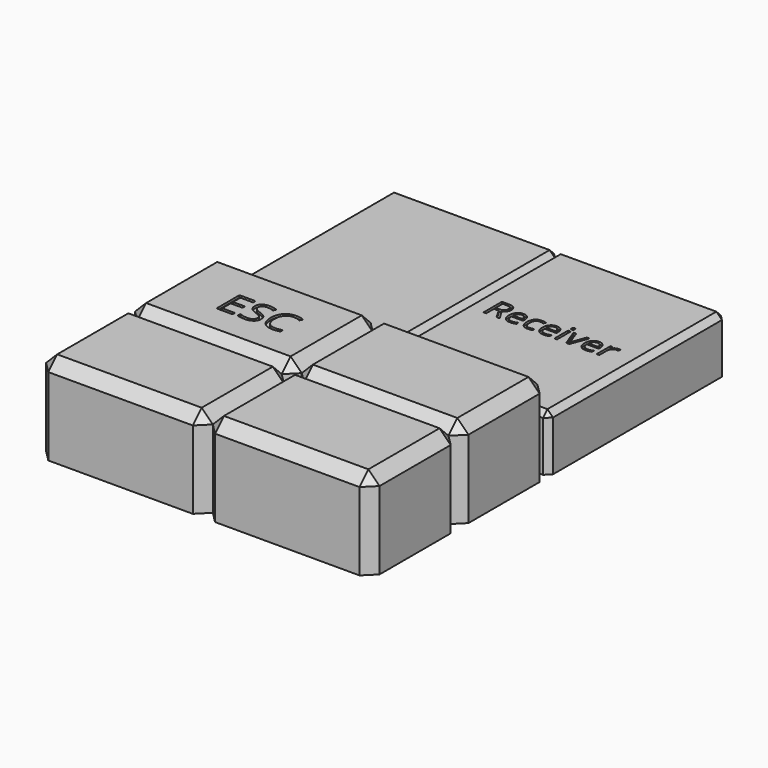
from build123d import *

# Parameters (mm, degrees)
F0_W            = 75
F0_H            = 50
F1_DEPTH        = 40
F2_SIZE         = 5
F5_DEPTH        = 25
F6_SIZE         = 2.5
F8_TEXT_SIZE    = 18.064936416
F9_DEPTH        = 1
F10_TEXT_SIZE   = 13.8888888889
F10_TEXT_SIZE_2 = 14.4519739681
F11_DEPTH       = 1


# Not quite as in the source:
# - Text() gives the source's letters only with a copy of the font that has no kerning and outlines rounded to 1/6400 em; it was checked with that copy


with BuildPart() as f1:
    # F0 (on Top) → F1 (new body)
    with BuildSketch(Plane.XY):
        with Locations((37.5, 25)):
            Rectangle(F0_W, F0_H)
    extrude(amount=F1_DEPTH)

    # F2
    f2_edges = [f1.edges().sort_by_distance(p)[0] for p in [
        (0, 0, 20),
        (75, 0, 20),
        (75, 50, 20),
        (0, 50, 20),
        (0, 25, 40),
        (37.5, 0, 40),
        (75, 25, 40),
        (37.5, 50, 40),
    ]]
    chamfer(f2_edges, length=F2_SIZE)

    # F3: F1 across face


with BuildPart() as f1_1:
    add(f1.part)
    add(f1.part.mirror(Plane(origin=(37.5, 50, 17.5), x_dir=(-1, 0, 0), z_dir=(0, 1, 0))))

    # F4 (on face) → F5 (join)
    with BuildSketch(Plane(origin=(0, 0, 0), x_dir=(1, 0, 0), z_dir=(0, 0, -1))):
        Polygon((5, -100), (0, -100), (0, -200), (75, -200), (75, -100), (70, -100), align=None)
    extrude(amount=-F5_DEPTH)

    # F6
    f6_edges = [f1_1.edges().sort_by_distance(p)[0] for p in [
        (75, 100, 12.5),
        (75, 200, 12.5),
        (0, 200, 12.5),
        (0, 100, 12.5),
        (0, 150, 25),
        (75, 150, 25),
        (37.5, 200, 25),
        (72.5, 100, 25),
        (2.5, 100, 25),
    ]]
    chamfer(f6_edges, length=F6_SIZE)

    # F7: F1 across face


with BuildPart() as f1_2:
    add(f1_1.part)
    add(f1_1.part.mirror(Plane(origin=(75, 150, 11.25), x_dir=(0, 1, 0), z_dir=(1, 0, 0))))

    # F8 (on face) → F9 (cut)
    with BuildSketch(Plane.XY.offset(40)):
        with Locations((25.1013506204, 67.2466233373)):
            Text('ESC', F8_TEXT_SIZE, font='Open Sans', text_align=(TextAlign.LEFT, TextAlign.BOTTOM))
    extrude(amount=-F9_DEPTH, mode=Mode.SUBTRACT)

    # F10 (on face) → F11 (cut)
    with BuildSketch(Plane.XY.offset(25)):
        with Locations((152.401474429, 218.4891363927)):
            Text('Reciever', F10_TEXT_SIZE, font='Open Sans', text_align=(TextAlign.LEFT, TextAlign.BOTTOM))
        with Locations((82.5675725937, 145.9966152906)):
            Text('Receiver', F10_TEXT_SIZE_2, font='Open Sans', text_align=(TextAlign.LEFT, TextAlign.BOTTOM))
    extrude(amount=-F11_DEPTH, mode=Mode.SUBTRACT)


solid = f1_2.part
